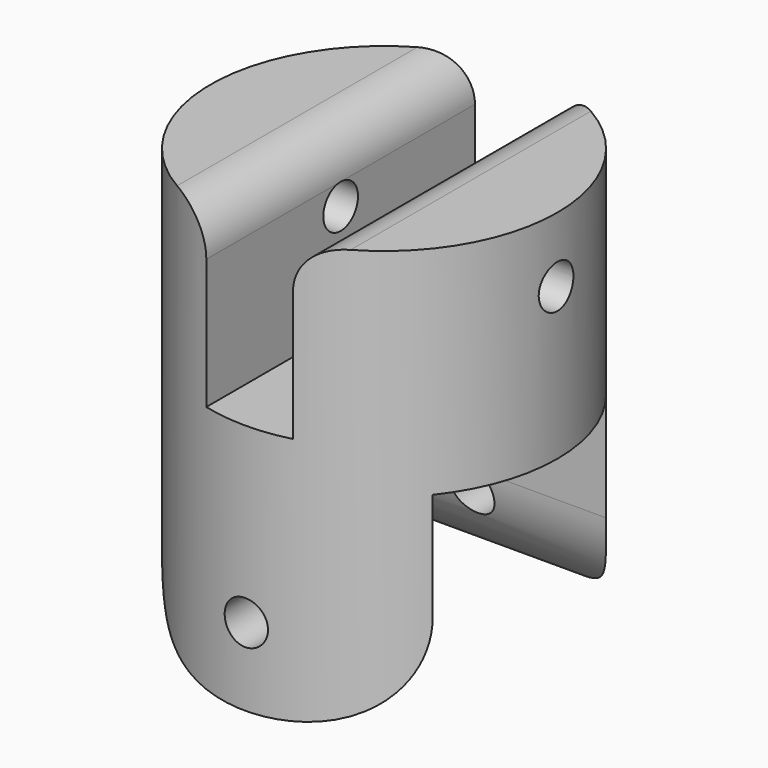
from build123d import *

# Parameters (mm, degrees)
F0_R        = 8
F1_DEPTH    = 20
F2_W        = 16
F2_H        = 10
F3_DEPTH    = 10
F4_T1_DEPTH = 37.4899959968
F5_R        = 1
F6_DEPTH    = 12.5
F8_DEPTH    = 8
F9_R        = 1
F10_DEPTH   = 12.5
F11_R       = 1.99999


# Not quite as in the source:
# - a fillet or chamfer that OpenCascade refuses, or shapes differently, is made with other operations: its cross-section is extruded or revolved along the edge and cut away or added
# - a fillet or chamfer is up to 0.001 mm smaller than in the source, because OpenCascade refuses the exact size


with BuildPart() as f1:
    # F0 (on Top) → F1 (new body)
    with BuildSketch(Plane.XY):
        Circle(F0_R)
    extrude(amount=F1_DEPTH)

    # F2 (on Top) → F3 (cut)
    with BuildSketch(Plane.XY):
        Rectangle(F2_W, F2_H)
    extrude(amount=F3_DEPTH, mode=Mode.SUBTRACT)

    # F4: fillet of radius 5 on 2 edges, made by hand

    # F4_s2 → F4_t1 (cut)
    with BuildSketch(Plane.YZ.offset(-18.7449979984)):
        with BuildLine():
            ThreePointArc((-10, 0), (-6.4644660941, 1.4644660941), (-5, 5))
            Line((-5, 5), (-5, 0))
            Line((-5, 0), (-10, 0))
        make_face()
        with BuildLine():
            ThreePointArc((10, 0), (6.4644660941, 1.4644660941), (5, 5))
            Line((5, 5), (5, 0))
            Line((5, 0), (10, 0))
        make_face()
    extrude(amount=F4_T1_DEPTH, mode=Mode.SUBTRACT)

    # F5 (on Front) → F6 (cut, symmetric)
    with BuildSketch(Plane.XZ):
        with Locations((0, 4)):
            Circle(F5_R)
    extrude(amount=F6_DEPTH, both=True, mode=Mode.SUBTRACT)

    # F7 (on face) → F8 (cut)
    with BuildSketch(Plane.XY.offset(20)):
        with BuildLine():
            ThreePointArc((2, 7.7459666924), (1.0080343399, 7.9362375701), (0, 8))
            ThreePointArc((0, 8), (-1.0080343399, 7.9362375701), (-2, 7.7459666924))
            Line((-2, 7.7459666924), (-2, -7.7459666924))
            ThreePointArc((-2, -7.7459666924), (-1.0080343399, -7.9362375701), (0, -8))
            ThreePointArc((0, -8), (1.0080343399, -7.9362375701), (2, -7.7459666924))
            Line((2, -7.7459666924), (2, 7.7459666924))
        make_face()
    extrude(amount=-F8_DEPTH, mode=Mode.SUBTRACT)

    # F9 (on Right) → F10 (cut, symmetric)
    with BuildSketch(Plane.YZ):
        with Locations((0, 17)):
            Circle(F9_R)
    extrude(amount=F10_DEPTH, both=True, mode=Mode.SUBTRACT)

    # F11 (radius 2 in the source; OpenCascade refuses exactly that, so slightly less here)
    f11_edges = [f1.edges().sort_by_distance(p)[0] for p in [
        (-2, 0, 20),
        (2, 0, 20),
    ]]
    fillet(f11_edges, radius=F11_R)


solid = f1.part
